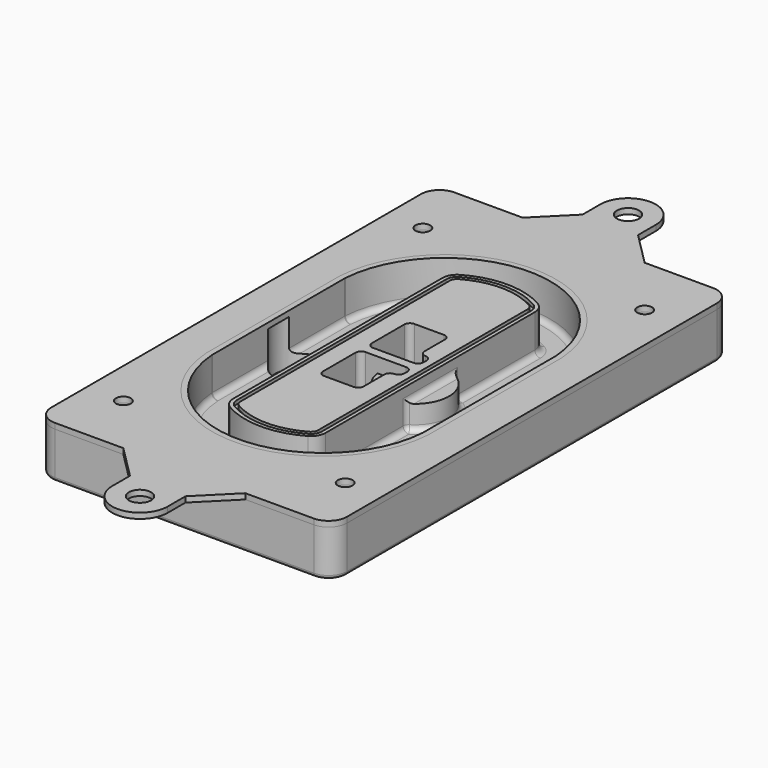
from build123d import *

# Parameters (mm, degrees)
F0_R      = 4
F1_DEPTH  = 25
F2_DEPTH  = 3
F3_DEPTH  = 18
F5_DEPTH  = 21
F6_DEPTH  = 2
F8_DEPTH  = 20
F9_DEPTH  = 16
F10_DEPTH = 25
F7_R      = 6
F7_R_2    = 4
F11_DEPTH = 6
F13_DEPTH = 9
F14_R     = 3
F15_R     = 2
F16_R     = 4
F16_R_2   = 6
F17_DEPTH = 3


with BuildPart() as f1:
    # F0 (on Top) → F1 (new body)
    with BuildSketch(Plane.XY):
        with BuildLine():
            ThreePointArc((-80, -125), (-77.0710678119, -132.0710678119), (-70, -135))
            Line((-70, -135), (70, -135))
            ThreePointArc((70, -135), (77.0710678119, -132.0710678119), (80, -125))
            Line((80, -125), (80, 125))
            ThreePointArc((80, 125), (77.0710678119, 132.0710678119), (70, 135))
            Line((70, 135), (-70, 135))
            ThreePointArc((-70, 135), (-77.0710678119, 132.0710678119), (-80, 125))
            Line((-80, 125), (-80, -125))
        make_face()
        with Locations((-60, -101.25)):
            Circle(F0_R, mode=Mode.SUBTRACT)
        with Locations((60, -101.25)):
            Circle(F0_R, mode=Mode.SUBTRACT)
        with Locations((-60, 101.25)):
            Circle(F0_R, mode=Mode.SUBTRACT)
        with BuildLine():
            ThreePointArc((-64, 44.6627429245), (-63.991269098, 45.1571001106), (-63.9650872818, 45.650840699))
            ThreePointArc((-63.9650872818, 45.650840699), (0, 105.25), (63.9650872818, 45.650840699))
            ThreePointArc((63.9650872818, 45.650840699), (63.991269098, 45.1571001106), (64, 44.6627429245))
            Line((64, 44.6627429245), (64, -44.6627429245))
            ThreePointArc((64, -44.6627429245), (63.991269098, -45.1571001106), (63.9650872818, -45.650840699))
            ThreePointArc((63.9650872818, -45.650840699), (0, -105.25), (-63.9650872818, -45.650840699))
            ThreePointArc((-63.9650872818, -45.650840699), (-63.991269098, -45.1571001106), (-64, -44.6627429245))
            Line((-64, -44.6627429245), (-64, 44.6627429245))
        make_face(mode=Mode.SUBTRACT)
        with Locations((60, 101.25)):
            Circle(F0_R, mode=Mode.SUBTRACT)
        with BuildLine():
            ThreePointArc((63.9650872818, 45.650840699), (0, 105.25), (-63.9650872818, 45.650840699))
            ThreePointArc((-63.9650872818, 45.650840699), (-63.991269098, 45.1571001106), (-64, 44.6627429245))
            Line((-64, 44.6627429245), (-64, -44.6627429245))
            ThreePointArc((-64, -44.6627429245), (-63.991269098, -45.1571001106), (-63.9650872818, -45.650840699))
            ThreePointArc((-63.9650872818, -45.650840699), (0, -105.25), (63.9650872818, -45.650840699))
            ThreePointArc((63.9650872818, -45.650840699), (63.991269098, -45.1571001106), (64, -44.6627429245))
            Line((64, -44.6627429245), (64, 44.6627429245))
            ThreePointArc((64, 44.6627429245), (63.991269098, 45.1571001106), (63.9650872818, 45.650840699))
        make_face()
        with BuildLine():
            Line((-60, -44.6627429245), (-60, 44.6627429245))
            ThreePointArc((-60, 44.6627429245), (-59.9937636414, 45.0158552003), (-59.9750623441, 45.3685270491))
            ThreePointArc((-59.9750623441, 45.3685270491), (0, 101.25), (59.9750623441, 45.3685270491))
            ThreePointArc((59.9750623441, 45.3685270491), (59.9937636414, 45.0158552003), (60, 44.6627429245))
            Line((60, 44.6627429245), (60, -44.6627429245))
            ThreePointArc((60, -44.6627429245), (59.9937636414, -45.0158552003), (59.9750623441, -45.3685270491))
            ThreePointArc((59.9750623441, -45.3685270491), (0, -101.25), (-59.9750623441, -45.3685270491))
            ThreePointArc((-59.9750623441, -45.3685270491), (-59.9937636414, -45.0158552003), (-60, -44.6627429245))
        make_face(mode=Mode.SUBTRACT)
        with BuildLine():
            ThreePointArc((-59.9750623441, 45.3685270491), (-59.9937636414, 45.0158552003), (-60, 44.6627429245))
            Line((-60, 44.6627429245), (-60, -44.6627429245))
            ThreePointArc((-60, -44.6627429245), (-59.9937636414, -45.0158552003), (-59.9750623441, -45.3685270491))
            ThreePointArc((-59.9750623441, -45.3685270491), (0, -101.25), (59.9750623441, -45.3685270491))
            ThreePointArc((59.9750623441, -45.3685270491), (59.9937636414, -45.0158552003), (60, -44.6627429245))
            Line((60, -44.6627429245), (60, 44.6627429245))
            ThreePointArc((60, 44.6627429245), (59.9937636414, 45.0158552003), (59.9750623441, 45.3685270491))
            ThreePointArc((59.9750623441, 45.3685270491), (0, 101.25), (-59.9750623441, 45.3685270491))
        make_face()
        with BuildLine():
            ThreePointArc((56.9825436409, 45.1567918117), (56.995634549, 44.9099215176), (57, 44.6627429245))
            Line((57, 44.6627429245), (57, -44.6627429245))
            ThreePointArc((57, -44.6627429245), (56.995634549, -44.9099215176), (56.9825436409, -45.1567918117))
            ThreePointArc((56.9825436409, -45.1567918117), (0, -98.25), (-56.9825436409, -45.1567918117))
            ThreePointArc((-56.9825436409, -45.1567918117), (-56.995634549, -44.9099215176), (-57, -44.6627429245))
            Line((-57, -44.6627429245), (-57, 44.6627429245))
            ThreePointArc((-57, 44.6627429245), (-56.995634549, 44.9099215176), (-56.9825436409, 45.1567918117))
            ThreePointArc((-56.9825436409, 45.1567918117), (0, 98.25), (56.9825436409, 45.1567918117))
        make_face(mode=Mode.SUBTRACT)
        with BuildLine():
            Line((57, -44.6627429245), (57, 44.6627429245))
            ThreePointArc((57, 44.6627429245), (56.995634549, 44.9099215176), (56.9825436409, 45.1567918117))
            ThreePointArc((56.9825436409, 45.1567918117), (0, 98.25), (-56.9825436409, 45.1567918117))
            ThreePointArc((-56.9825436409, 45.1567918117), (-56.995634549, 44.9099215176), (-57, 44.6627429245))
            Line((-57, 44.6627429245), (-57, -44.6627429245))
            ThreePointArc((-57, -44.6627429245), (-56.995634549, -44.9099215176), (-56.9825436409, -45.1567918117))
            ThreePointArc((-56.9825436409, -45.1567918117), (0, -98.25), (56.9825436409, -45.1567918117))
            ThreePointArc((56.9825436409, -45.1567918117), (56.995634549, -44.9099215176), (57, -44.6627429245))
        make_face()
    extrude(amount=-F1_DEPTH)

    # F0 (on Top) → F2 (join)
    with BuildSketch(Plane.XY):
        with BuildLine():
            ThreePointArc((-59.9750623441, 45.3685270491), (-59.9937636414, 45.0158552003), (-60, 44.6627429245))
            Line((-60, 44.6627429245), (-60, -44.6627429245))
            ThreePointArc((-60, -44.6627429245), (-59.9937636414, -45.0158552003), (-59.9750623441, -45.3685270491))
            ThreePointArc((-59.9750623441, -45.3685270491), (0, -101.25), (59.9750623441, -45.3685270491))
            ThreePointArc((59.9750623441, -45.3685270491), (59.9937636414, -45.0158552003), (60, -44.6627429245))
            Line((60, -44.6627429245), (60, 44.6627429245))
            ThreePointArc((60, 44.6627429245), (59.9937636414, 45.0158552003), (59.9750623441, 45.3685270491))
            ThreePointArc((59.9750623441, 45.3685270491), (0, 101.25), (-59.9750623441, 45.3685270491))
        make_face()
        with BuildLine():
            ThreePointArc((56.9825436409, 45.1567918117), (56.995634549, 44.9099215176), (57, 44.6627429245))
            Line((57, 44.6627429245), (57, -44.6627429245))
            ThreePointArc((57, -44.6627429245), (56.995634549, -44.9099215176), (56.9825436409, -45.1567918117))
            ThreePointArc((56.9825436409, -45.1567918117), (0, -98.25), (-56.9825436409, -45.1567918117))
            ThreePointArc((-56.9825436409, -45.1567918117), (-56.995634549, -44.9099215176), (-57, -44.6627429245))
            Line((-57, -44.6627429245), (-57, 44.6627429245))
            ThreePointArc((-57, 44.6627429245), (-56.995634549, 44.9099215176), (-56.9825436409, 45.1567918117))
            ThreePointArc((-56.9825436409, 45.1567918117), (0, 98.25), (56.9825436409, 45.1567918117))
        make_face(mode=Mode.SUBTRACT)
    extrude(amount=F2_DEPTH)

    # F0 (on Top) → F3 (cut)
    with BuildSketch(Plane.XY):
        with BuildLine():
            Line((57, -44.6627429245), (57, 44.6627429245))
            ThreePointArc((57, 44.6627429245), (56.995634549, 44.9099215176), (56.9825436409, 45.1567918117))
            ThreePointArc((56.9825436409, 45.1567918117), (0, 98.25), (-56.9825436409, 45.1567918117))
            ThreePointArc((-56.9825436409, 45.1567918117), (-56.995634549, 44.9099215176), (-57, 44.6627429245))
            Line((-57, 44.6627429245), (-57, -44.6627429245))
            ThreePointArc((-57, -44.6627429245), (-56.995634549, -44.9099215176), (-56.9825436409, -45.1567918117))
            ThreePointArc((-56.9825436409, -45.1567918117), (0, -98.25), (56.9825436409, -45.1567918117))
            ThreePointArc((56.9825436409, -45.1567918117), (56.995634549, -44.9099215176), (57, -44.6627429245))
        make_face()
    extrude(amount=-F3_DEPTH, mode=Mode.SUBTRACT)

    # F4 (on face) → F5 (join, through all)
    with BuildSketch(Plane.XY.offset(3)):
        with BuildLine():
            ThreePointArc((-25, -70.7141132851), (-23.9239722661, -74.7214325959), (-20.9853479853, -77.6507552274))
            ThreePointArc((-20.9853479853, -77.6507552274), (0, -83.25), (20.9853479853, -77.6507552274))
            ThreePointArc((20.9853479853, -77.6507552274), (23.9239722661, -74.7214325959), (25, -70.7141132851))
            Line((25, -70.7141132851), (25, 70.7141132851))
            ThreePointArc((25, 70.7141132851), (23.9239722661, 74.7214325959), (20.9853479853, 77.6507552274))
            ThreePointArc((20.9853479853, 77.6507552274), (0, 83.25), (-20.9853479853, 77.6507552274))
            ThreePointArc((-20.9853479853, 77.6507552274), (-23.9239722661, 74.7214325959), (-25, 70.7141132851))
            Line((-25, 70.7141132851), (-25, -70.7141132851))
        make_face()
        with BuildLine():
            ThreePointArc((19.989010989, 75.9165947419), (22.1929791996, 73.7196027682), (23, 70.7141132851))
            Line((23, 70.7141132851), (23, -70.7141132851))
            ThreePointArc((23, -70.7141132851), (22.1929791996, -73.7196027682), (19.989010989, -75.9165947419))
            ThreePointArc((19.989010989, -75.9165947419), (0, -81.25), (-19.989010989, -75.9165947419))
            ThreePointArc((-19.989010989, -75.9165947419), (-22.1929791996, -73.7196027682), (-23, -70.7141132851))
            Line((-23, -70.7141132851), (-23, 70.7141132851))
            ThreePointArc((-23, 70.7141132851), (-22.1929791996, 73.7196027682), (-19.989010989, 75.9165947419))
            ThreePointArc((-19.989010989, 75.9165947419), (0, 81.25), (19.989010989, 75.9165947419))
        make_face(mode=Mode.SUBTRACT)
        with BuildLine():
            Line((23, -70.7141132851), (23, 70.7141132851))
            ThreePointArc((23, 70.7141132851), (22.1929791996, 73.7196027682), (19.989010989, 75.9165947419))
            ThreePointArc((19.989010989, 75.9165947419), (0, 81.25), (-19.989010989, 75.9165947419))
            ThreePointArc((-19.989010989, 75.9165947419), (-22.1929791996, 73.7196027682), (-23, 70.7141132851))
            Line((-23, 70.7141132851), (-23, -70.7141132851))
            ThreePointArc((-23, -70.7141132851), (-22.1929791996, -73.7196027682), (-19.989010989, -75.9165947419))
            ThreePointArc((-19.989010989, -75.9165947419), (0, -81.25), (19.989010989, -75.9165947419))
            ThreePointArc((19.989010989, -75.9165947419), (22.1929791996, -73.7196027682), (23, -70.7141132851))
        make_face()
        with BuildLine():
            ThreePointArc((18.9926739927, 74.1824342563), (20.461986133, 72.7177729405), (21, 70.7141132851))
            Line((21, 70.7141132851), (21, -70.7141132851))
            ThreePointArc((21, -70.7141132851), (20.461986133, -72.7177729405), (18.9926739927, -74.1824342563))
            ThreePointArc((18.9926739927, -74.1824342563), (0, -79.25), (-18.9926739927, -74.1824342563))
            ThreePointArc((-18.9926739927, -74.1824342563), (-20.461986133, -72.7177729405), (-21, -70.7141132851))
            Line((-21, -70.7141132851), (-21, 70.7141132851))
            ThreePointArc((-21, 70.7141132851), (-20.461986133, 72.7177729405), (-18.9926739927, 74.1824342563))
            ThreePointArc((-18.9926739927, 74.1824342563), (0, 79.25), (18.9926739927, 74.1824342563))
        make_face(mode=Mode.SUBTRACT)
        with BuildLine():
            Line((21, -70.7141132851), (21, 70.7141132851))
            ThreePointArc((21, 70.7141132851), (20.461986133, 72.7177729405), (18.9926739927, 74.1824342563))
            ThreePointArc((18.9926739927, 74.1824342563), (0, 79.25), (-18.9926739927, 74.1824342563))
            ThreePointArc((-18.9926739927, 74.1824342563), (-20.461986133, 72.7177729405), (-21, 70.7141132851))
            Line((-21, 70.7141132851), (-21, -70.7141132851))
            ThreePointArc((-21, -70.7141132851), (-20.461986133, -72.7177729405), (-18.9926739927, -74.1824342563))
            ThreePointArc((-18.9926739927, -74.1824342563), (0, -79.25), (18.9926739927, -74.1824342563))
            ThreePointArc((18.9926739927, -74.1824342563), (20.461986133, -72.7177729405), (21, -70.7141132851))
        make_face()
        with BuildLine():
            Line((-8, -2.5), (14, -2.5))
            ThreePointArc((14, -2.5), (16.1213203436, -3.3786796564), (17, -5.5))
            Line((17, -5.5), (17, -7.5))
            ThreePointArc((17, -7.5), (16.1213203436, -9.6213203436), (14, -10.5))
            ThreePointArc((14, -10.5), (11.8786796564, -11.3786796564), (11, -13.5))
            Line((11, -13.5), (11, -27.5))
            ThreePointArc((11, -27.5), (10.1213203436, -29.6213203436), (8, -30.5))
            Line((8, -30.5), (-8, -30.5))
            ThreePointArc((-8, -30.5), (-10.1213203436, -29.6213203436), (-11, -27.5))
            Line((-11, -27.5), (-11, -5.5))
            ThreePointArc((-11, -5.5), (-10.1213203436, -3.3786796564), (-8, -2.5))
        make_face(mode=Mode.SUBTRACT)
        with BuildLine():
            ThreePointArc((-8, 2.5), (-10.1213203436, 3.3786796564), (-11, 5.5))
            Line((-11, 5.5), (-11, 27.5))
            ThreePointArc((-11, 27.5), (-10.1213203436, 29.6213203436), (-8, 30.5))
            Line((-8, 30.5), (8, 30.5))
            ThreePointArc((8, 30.5), (10.1213203436, 29.6213203436), (11, 27.5))
            Line((11, 27.5), (11, 13.5))
            ThreePointArc((11, 13.5), (11.8786796564, 11.3786796564), (14, 10.5))
            ThreePointArc((14, 10.5), (16.1213203436, 9.6213203436), (17, 7.5))
            Line((17, 7.5), (17, 5.5))
            ThreePointArc((17, 5.5), (16.1213203436, 3.3786796564), (14, 2.5))
            Line((14, 2.5), (-8, 2.5))
        make_face(mode=Mode.SUBTRACT)
    extrude(amount=-F5_DEPTH)

    # F4 (on face) → F6 (cut)
    with BuildSketch(Plane.XY.offset(3)):
        with BuildLine():
            Line((23, -70.7141132851), (23, 70.7141132851))
            ThreePointArc((23, 70.7141132851), (22.1929791996, 73.7196027682), (19.989010989, 75.9165947419))
            ThreePointArc((19.989010989, 75.9165947419), (0, 81.25), (-19.989010989, 75.9165947419))
            ThreePointArc((-19.989010989, 75.9165947419), (-22.1929791996, 73.7196027682), (-23, 70.7141132851))
            Line((-23, 70.7141132851), (-23, -70.7141132851))
            ThreePointArc((-23, -70.7141132851), (-22.1929791996, -73.7196027682), (-19.989010989, -75.9165947419))
            ThreePointArc((-19.989010989, -75.9165947419), (0, -81.25), (19.989010989, -75.9165947419))
            ThreePointArc((19.989010989, -75.9165947419), (22.1929791996, -73.7196027682), (23, -70.7141132851))
        make_face()
        with BuildLine():
            ThreePointArc((18.9926739927, 74.1824342563), (20.461986133, 72.7177729405), (21, 70.7141132851))
            Line((21, 70.7141132851), (21, -70.7141132851))
            ThreePointArc((21, -70.7141132851), (20.461986133, -72.7177729405), (18.9926739927, -74.1824342563))
            ThreePointArc((18.9926739927, -74.1824342563), (0, -79.25), (-18.9926739927, -74.1824342563))
            ThreePointArc((-18.9926739927, -74.1824342563), (-20.461986133, -72.7177729405), (-21, -70.7141132851))
            Line((-21, -70.7141132851), (-21, 70.7141132851))
            ThreePointArc((-21, 70.7141132851), (-20.461986133, 72.7177729405), (-18.9926739927, 74.1824342563))
            ThreePointArc((-18.9926739927, 74.1824342563), (0, 79.25), (18.9926739927, 74.1824342563))
        make_face(mode=Mode.SUBTRACT)
    extrude(amount=-F6_DEPTH, mode=Mode.SUBTRACT)

    # F7 (on face) → F8 (join)
    with BuildSketch(Plane(origin=(0, 0, -25), x_dir=(1, 0, 0), z_dir=(0, 0, -1))):
        with BuildLine():
            ThreePointArc((3.28842436, 0), (16.7567035675, 13.4682792075), (30.224982775, 0))
            Line((30.224982775, 0), (35.224982775, 0))
            ThreePointArc((35.224982775, 0), (16.7567035675, 18.4682792075), (-1.71157564, 0))
            Line((-1.71157564, 0), (3.28842436, 0))
        make_face()
        with BuildLine():
            Line((3.28842436, 0), (30.224982775, 0))
            ThreePointArc((30.224982775, 0), (16.7567035675, 13.4682792075), (3.28842436, 0))
        make_face()
        with BuildLine():
            ThreePointArc((3.28842436, 0), (16.7567035675, -13.4682792075), (30.224982775, 0))
            Line((30.224982775, 0), (3.28842436, 0))
        make_face()
        with BuildLine():
            Line((35.224982775, 0), (30.224982775, 0))
            ThreePointArc((30.224982775, 0), (16.7567035675, -13.4682792075), (3.28842436, 0))
            Line((3.28842436, 0), (-1.71157564, 0))
            ThreePointArc((-1.71157564, 0), (16.7567035675, -18.4682792075), (35.224982775, 0))
        make_face()
    extrude(amount=-F8_DEPTH)

    # F7 (on face) → F9 (cut)
    with BuildSketch(Plane(origin=(0, 0, -25), x_dir=(1, 0, 0), z_dir=(0, 0, -1))):
        with BuildLine():
            Line((3.28842436, 0), (30.224982775, 0))
            ThreePointArc((30.224982775, 0), (16.7567035675, 13.4682792075), (3.28842436, 0))
        make_face()
        with BuildLine():
            ThreePointArc((3.28842436, 0), (16.7567035675, -13.4682792075), (30.224982775, 0))
            Line((30.224982775, 0), (3.28842436, 0))
        make_face()
    extrude(amount=-F9_DEPTH, mode=Mode.SUBTRACT)

    # F7 (on face) → F10 (cut)
    with BuildSketch(Plane(origin=(0, 0, -25), x_dir=(1, 0, 0), z_dir=(0, 0, -1))):
        with BuildLine():
            Line((-59.0318229325, 0), (-32.0952645175, 0))
            ThreePointArc((-32.0952645175, 0), (-45.563543725, 13.4682792075), (-59.0318229325, 0))
        make_face()
        with BuildLine():
            ThreePointArc((-59.0318229325, 0), (-45.563543725, -13.4682792075), (-32.0952645175, 0))
            Line((-32.0952645175, 0), (-59.0318229325, 0))
        make_face()
    extrude(amount=-F10_DEPTH, mode=Mode.SUBTRACT)

    # F7 (on face) → F11 (cut)
    with BuildSketch(Plane(origin=(0, 0, -25), x_dir=(1, 0, 0), z_dir=(0, 0, -1))):
        with Locations((60, -101.25)):
            Circle(F7_R)
        with Locations((60, -101.25)):
            Circle(F7_R_2, mode=Mode.SUBTRACT)
        with Locations((-60, -101.25)):
            Circle(F7_R)
        with Locations((-60, -101.25)):
            Circle(F7_R_2, mode=Mode.SUBTRACT)
        with Locations((-60, 101.25)):
            Circle(F7_R)
        with Locations((-60, 101.25)):
            Circle(F7_R_2, mode=Mode.SUBTRACT)
        with Locations((60, 101.25)):
            Circle(F7_R)
        with Locations((60, 101.25)):
            Circle(F7_R_2, mode=Mode.SUBTRACT)
    extrude(amount=-F11_DEPTH, mode=Mode.SUBTRACT)

    # F12 (on face) → F13 (cut, through all)
    with BuildSketch(Plane(origin=(0, 0, -9), x_dir=(1, 0, 0), z_dir=(0, 0, -1))):
        with BuildLine():
            Line((11, 13.5), (11, 17.5481537753))
            ThreePointArc((11, 17.5481537753), (2.5696536419, 11.8239143813), (-1.5415842455, 2.5))
            Line((-1.5415842455, 2.5), (3.5224848595, 2.5))
            ThreePointArc((3.5224848595, 2.5), (6.1857188154, 8.3455872281), (11.2536447004, 12.2927168648))
            ThreePointArc((11.2536447004, 12.2927168648), (11.0640958889, 12.8831798879), (11, 13.5))
        make_face()
        with BuildLine():
            ThreePointArc((11.2536447004, -12.2927168648), (6.1857188154, -8.3455872281), (3.5224848595, -2.5))
            Line((3.5224848595, -2.5), (-1.5415842455, -2.5))
            ThreePointArc((-1.5415842455, -2.5), (2.5696536419, -11.8239143813), (11, -17.5481537753))
            Line((11, -17.5481537753), (11, -13.5))
            ThreePointArc((11, -13.5), (11.0640958889, -12.8831798879), (11.2536447004, -12.2927168648))
        make_face()
        with BuildLine():
            ThreePointArc((11.2536447004, 12.2927168648), (6.1857188154, 8.3455872281), (3.5224848595, 2.5))
            Line((3.5224848595, 2.5), (14, 2.5))
            ThreePointArc((14, 2.5), (16.1213203436, 3.3786796564), (17, 5.5))
            Line((17, 5.5), (17, 7.5))
            ThreePointArc((17, 7.5), (16.1213203436, 9.6213203436), (14, 10.5))
            ThreePointArc((14, 10.5), (12.3601599782, 10.9878446101), (11.2536447004, 12.2927168648))
        make_face()
        with BuildLine():
            Line((14, -2.5), (3.5224848595, -2.5))
            ThreePointArc((3.5224848595, -2.5), (6.1857188154, -8.3455872281), (11.2536447004, -12.2927168648))
            ThreePointArc((11.2536447004, -12.2927168648), (12.3601599782, -10.9878446101), (14, -10.5))
            ThreePointArc((14, -10.5), (16.1213203436, -9.6213203436), (17, -7.5))
            Line((17, -7.5), (17, -5.5))
            ThreePointArc((17, -5.5), (16.1213203436, -3.3786796564), (14, -2.5))
        make_face()
    extrude(amount=F13_DEPTH, mode=Mode.SUBTRACT)

    # F14
    f14_edges = [f1.edges().sort_by_distance(p)[0] for p in [
        (-57, -25.888126, -18),
        (-57, 25.888126, -18),
        (25, 0, -5),
        (25, 16.526506, -11.5),
        (25, -16.526506, -11.5),
        (25, -43.62031, -18),
        (35.224983, 0, -18),
    ]]
    fillet(f14_edges, radius=F14_R)

    # F15
    f15_edges = [f1.edges().sort_by_distance(p)[0] for p in [
        (0, -135, -25),
    ]]
    fillet(f15_edges, radius=F15_R)


with BuildPart() as f17:
    # F16 (on face) → F17 (new body, through all)
    with BuildSketch(Plane.XY):
        with BuildLine():
            Line((-33, 135), (-70, 135))
            ThreePointArc((-70, 135), (-77.0710678119, 132.0710678119), (-80, 125))
            Line((-80, 125), (-80, -125))
            ThreePointArc((-80, -125), (-77.0710678119, -132.0710678119), (-70, -135))
            Line((-70, -135), (-33, -135))
            Line((-33, -135), (33, -135))
            Line((33, -135), (70, -135))
            ThreePointArc((70, -135), (77.0710678119, -132.0710678119), (80, -125))
            Line((80, -125), (80, 125))
            ThreePointArc((80, 125), (77.0710678119, 132.0710678119), (70, 135))
            Line((70, 135), (33, 135))
            Line((33, 135), (-33, 135))
        make_face()
        with Locations((-60, -101.25)):
            Circle(F16_R, mode=Mode.SUBTRACT)
        with Locations((60, -101.25)):
            Circle(F16_R, mode=Mode.SUBTRACT)
        with Locations((-60, 101.25)):
            Circle(F16_R, mode=Mode.SUBTRACT)
        with BuildLine():
            ThreePointArc((-60, 44.6627429245), (-59.9937636414, 45.0158552003), (-59.9750623441, 45.3685270491))
            ThreePointArc((-59.9750623441, 45.3685270491), (0, 101.25), (59.9750623441, 45.3685270491))
            ThreePointArc((59.9750623441, 45.3685270491), (59.9937636414, 45.0158552003), (60, 44.6627429245))
            Line((60, 44.6627429245), (60, -44.6627429245))
            ThreePointArc((60, -44.6627429245), (59.9937636414, -45.0158552003), (59.9750623441, -45.3685270491))
            ThreePointArc((59.9750623441, -45.3685270491), (0, -101.25), (-59.9750623441, -45.3685270491))
            ThreePointArc((-59.9750623441, -45.3685270491), (-59.9937636414, -45.0158552003), (-60, -44.6627429245))
            Line((-60, -44.6627429245), (-60, 44.6627429245))
        make_face(mode=Mode.SUBTRACT)
        with Locations((60, 101.25)):
            Circle(F16_R, mode=Mode.SUBTRACT)
        with BuildLine():
            Line((-15, 153), (-33, 135))
            Line((-33, 135), (33, 135))
            Line((33, 135), (15, 153))
            Line((15, 153), (15, 165))
            ThreePointArc((15, 165), (0, 180), (-15, 165))
            Line((-15, 165), (-15, 153))
        make_face()
        with Locations((0, 165)):
            Circle(F16_R_2, mode=Mode.SUBTRACT)
        with BuildLine():
            Line((33, -135), (-33, -135))
            Line((-33, -135), (-15, -153))
            Line((-15, -153), (-15, -165))
            ThreePointArc((-15, -165), (0, -180), (15, -165))
            Line((15, -165), (15, -153))
            Line((15, -153), (33, -135))
        make_face()
        with Locations((0, -165)):
            Circle(F16_R_2, mode=Mode.SUBTRACT)
    extrude(amount=F17_DEPTH)


solid = Compound([f1.part, f17.part])
